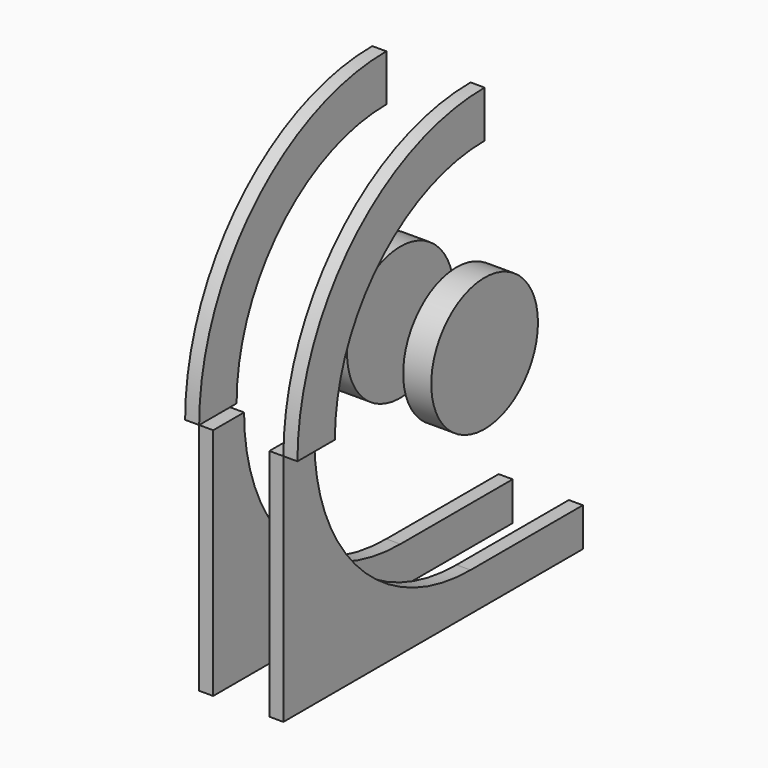
from build123d import *

# Parameters (mm, degrees)
F4_R      = 60.325
F5_DEPTH  = 25.4
F4_W      = 127
F4_H      = 34.925
F6_DEPTH  = 12.7
F7_DEPTH  = 12.7
F10_DEPTH = 12.7


# Not quite as in the source:
# - a variable given as a bare number and used for a length is read in inches; the dataset says mm whatever the document's units were


with BuildPart() as f5:
    # F4 (on offset) → F5 (new body)
    with BuildSketch(Plane.YZ.offset(25.4)):
        with Locations((0, 211.6328)):
            Circle(F4_R)
    extrude(amount=F5_DEPTH)


with BuildPart() as f6:
    # F4 (on offset) → F6 (new body)
    with BuildSketch(Plane.YZ.offset(25.4)):
        with BuildLine():
            ThreePointArc((-211.6328, 211.6328), (-149.6469880015, 61.9858119985), (0, 0))
            Line((0, 0), (0, 34.925))
            ThreePointArc((0, 34.925), (-124.9512836686, 86.6815163314), (-176.7078, 211.6328))
            Line((-176.7078, 211.6328), (-211.6328, 211.6328))
        make_face()
        with Locations((63.5, 17.4625)):
            Rectangle(F4_W, F4_H)
    extrude(amount=F6_DEPTH)

    # F4 (on offset) → F7 (join)
    with BuildSketch(Plane.YZ.offset(25.4)):
        with BuildLine():
            Line((-211.6328, 0), (0, 0))
            ThreePointArc((0, 0), (-149.6469880015, 61.9858119985), (-211.6328, 211.6328))
            Line((-211.6328, 211.6328), (-211.6328, 0))
        make_face()
    extrude(amount=F7_DEPTH)


with BuildPart() as f10:
    # F9 (on offset) → F10 (new body)
    with BuildSketch(Plane.YZ.offset(38.1)):
        with BuildLine():
            ThreePointArc((-169.3164, 211.6328), (-119.7247746061, 331.3575746061), (0, 380.9492))
            Line((0, 380.9492), (0, 423.2656))
            ThreePointArc((0, 423.2656), (-149.6469880015, 361.2797880015), (-211.6328, 211.6328))
            Line((-211.6328, 211.6328), (-169.3164, 211.6328))
        make_face()
    extrude(amount=F10_DEPTH)


with BuildPart() as f11_1:
    # F11: instance of F10
    add(f10.part.mirror(Plane.YZ))


with BuildPart() as f11_2:
    # F11: instance of F5
    add(f5.part.mirror(Plane.YZ))


with BuildPart() as f11_3:
    # F11: instance of F6
    add(f6.part.mirror(Plane.YZ))


solid = Compound([f5.part, f6.part, f10.part, f11_1.part, f11_2.part, f11_3.part])
